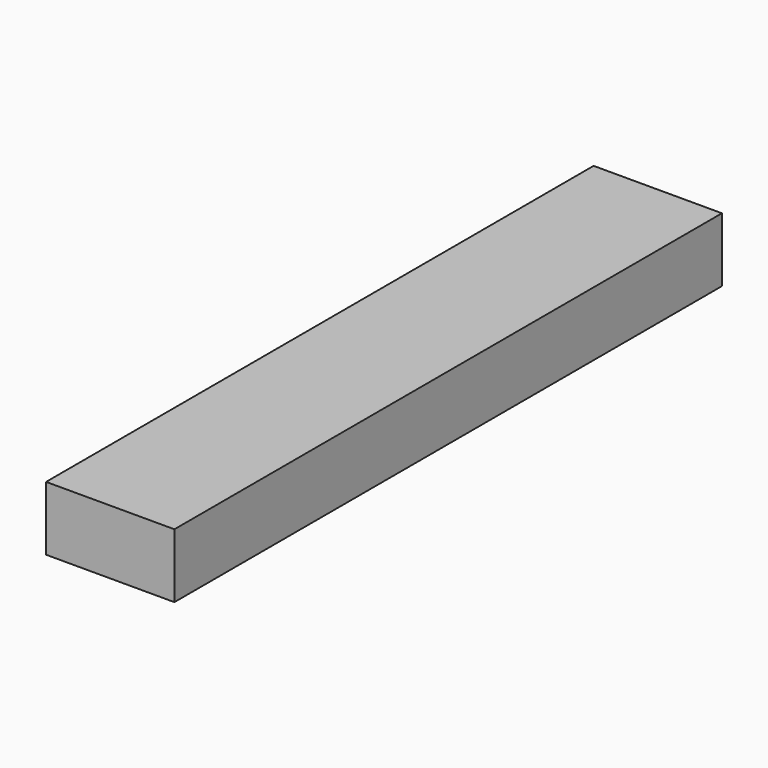
from build123d import *

# Parameters (mm, degrees)
F0_W     = 38.1
F0_H     = 203.2
F1_DEPTH = 19.05


# Not quite as in the source:
# - a length typed as a fraction of an inch, garbled in the dataset ("3 / 203.2 mm" for 3/8 in), is restored


with BuildPart() as f1:
    # F0 (on Top) → F1 (new body)
    with BuildSketch(Plane.XY):
        with Locations((-13.9456205746, 101.6)):
            Rectangle(F0_W, F0_H)
    extrude(amount=F1_DEPTH)


solid = f1.part
